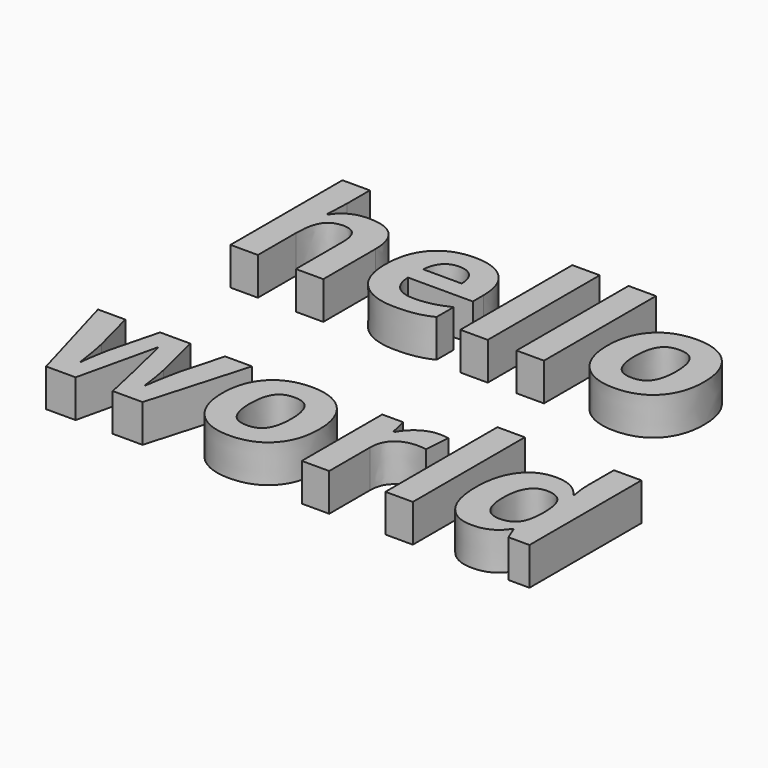
from build123d import *

# Parameters (mm, degrees)
F0_TEXT_SIZE = 124.2379347483
F1_DEPTH     = 25.4


# Not quite as in the source:
# - Text() gives the source's letters only with a copy of the font that has no kerning and outlines rounded to 1/6400 em; it was checked with that copy


with BuildPart() as f1:
    # F0 (on Top) → F1 (new body)
    with BuildSketch(Plane.XY):
        with Locations((-66.5969252586, -39.156422019)):
            Text('hello', F0_TEXT_SIZE, font='Open Sans', font_style=FontStyle.BOLD, text_align=(TextAlign.LEFT, TextAlign.BOTTOM))
        with Locations((-66.5969252586, -208.1200132767)):
            Text('world', F0_TEXT_SIZE, font='Open Sans', font_style=FontStyle.BOLD, text_align=(TextAlign.LEFT, TextAlign.BOTTOM))
    extrude(amount=F1_DEPTH)


solid = f1.part
